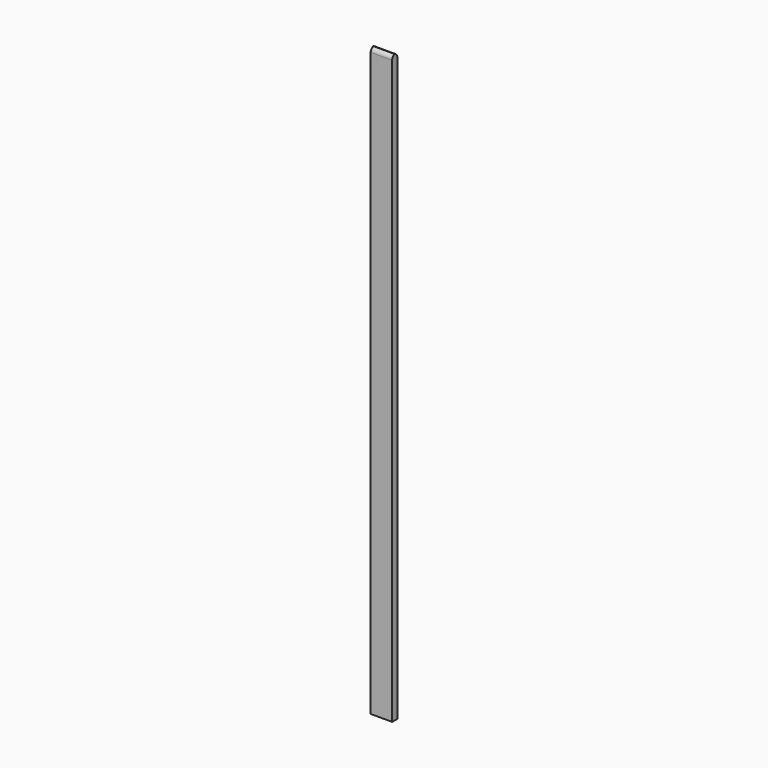
from build123d import *

# Parameters (mm, degrees)
F0_W        = 63.5
F0_H        = 1739.9
F1_DEPTH    = 19.05
F2_T1_DEPTH = 127


# Not quite as in the source:
# - a fillet or chamfer that OpenCascade refuses, or shapes differently, is made with other operations: its cross-section is extruded or revolved along the edge and cut away or added


with BuildPart() as f1:
    # F0 (on Front) → F1 (new body)
    with BuildSketch(Plane.XZ):
        Rectangle(F0_W, F0_H)
    extrude(amount=F1_DEPTH)

    # F2: fillet of radius 12.7 on 2 edges, made by hand

    # F2_s2 → F2_t1 (cut)
    with BuildSketch(Plane.YZ.offset(-63.5)):
        with BuildLine():
            ThreePointArc((-6.35, 869.95), (-15.3302561211, 866.2302561211), (-19.05, 857.25))
            Line((-19.05, 857.25), (-19.05, 869.95))
            Line((-19.05, 869.95), (-6.35, 869.95))
        make_face()
        with BuildLine():
            ThreePointArc((-12.7, 869.95), (-3.7197438789, 866.2302561211), (0, 857.25))
            Line((0, 857.25), (0, 869.95))
            Line((0, 869.95), (-12.7, 869.95))
        make_face()
    extrude(amount=F2_T1_DEPTH, mode=Mode.SUBTRACT)


solid = f1.part
